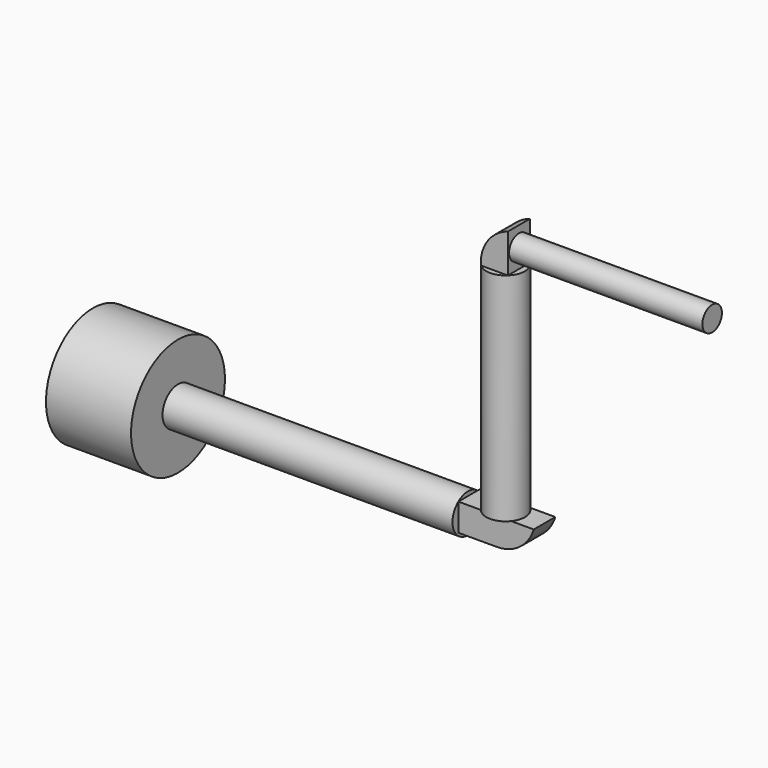
from build123d import *

# Parameters (mm, degrees)
F0_R         = 2.54
F1_DEPTH     = 38.1
F2_W         = 3.5423064731
F2_H         = 3.6002054004
F3_DEPTH     = 9.906
F4_T1_DEPTH  = 27.8407673004
F5_R         = 2.54
F6_DEPTH     = 28.448
F0_R_2       = 7.7136033571
F7_DEPTH     = 11.176
F9_DEPTH     = 5.08
F10_T1_DEPTH = 27.8075265616
F11_R        = 1.605342172
F12_DEPTH    = 25.4


# Not quite as in the source:
# - a fillet or chamfer that OpenCascade refuses, or shapes differently, is made with other operations: its cross-section is extruded or revolved along the edge and cut away or added


with BuildPart() as f1:
    # F0 (on Right) → F1 (new body)
    with BuildSketch(Plane.YZ):
        with Locations((-112.0406836271, 54.1470609605)):
            Circle(F0_R)
    extrude(amount=F1_DEPTH)

    # F2 (on face) → F3 (join)
    with BuildSketch(Plane.YZ.offset(38.1)):
        with Locations((-111.8464542239, 54.3381667436)):
            Rectangle(F2_W, F2_H)
    extrude(amount=F3_DEPTH)

    # F4: fillet of radius 5.08 on 1 edges, made by hand

    # F4_s2 → F4_t1 (cut)
    with BuildSketch(Plane.XZ.offset(97.9260705737)):
        with BuildLine():
            ThreePointArc((43.1463078345, 52.5380640434), (46.1702988592, 53.5361676357), (48.006, 56.1382694438))
            Line((48.006, 56.1382694438), (48.006, 52.5380640434))
            Line((48.006, 52.5380640434), (43.1463078345, 52.5380640434))
        make_face()
    extrude(amount=F4_T1_DEPTH, mode=Mode.SUBTRACT)

    # F5 (on face) → F6 (join)
    with BuildSketch(Plane.XY.offset(56.1382694438)):
        with Locations((43.053, -112.0406836271)):
            Circle(F5_R)
    extrude(amount=F6_DEPTH)

    # F8 (on face) → F9 (join)
    with BuildSketch(Plane.XY.offset(84.5862694438)):
        with BuildLine():
            Line((44.8093679455, -110.2645377603), (41.2372616213, -110.2645377603))
            Line((41.2372616213, -110.2645377603), (41.2372616213, -113.8168294939))
            ThreePointArc((41.2372616213, -113.8168294939), (41.2667054502, -113.8464388103), (41.2966320545, -113.8755600916))
            Line((41.2966320545, -113.8755600916), (44.8093679455, -113.8755600916))
            Line((44.8093679455, -113.8755600916), (44.8093679455, -110.2645377603))
        make_face()
    extrude(amount=F9_DEPTH)

    # F10: fillet of radius 5.08 on 1 edges, made by hand

    # F10_s2 → F10_t1 (cut)
    with BuildSketch(Plane.XZ.offset(98.1369203463)):
        with BuildLine():
            ThreePointArc((41.2372616213, 84.8152224782), (42.2266320932, 87.8273894828), (44.8093679455, 89.6662694438))
            Line((44.8093679455, 89.6662694438), (41.2372616213, 89.6662694438))
            Line((41.2372616213, 89.6662694438), (41.2372616213, 84.8152224782))
        make_face()
    extrude(amount=F10_T1_DEPTH, mode=Mode.SUBTRACT)

    # F11 (on face) → F12 (join)
    with BuildSketch(Plane.YZ.offset(44.8093679455)):
        with Locations((-112.070048926, 87.1262694438)):
            Circle(F11_R)
    extrude(amount=F12_DEPTH)


with BuildPart() as f7:
    # F0 (on Right) → F7 (new body)
    with BuildSketch(Plane.YZ):
        with Locations((-112.0406836271, 54.1470609605)):
            Circle(F0_R_2)
        with Locations((-112.0406836271, 54.1470609605)):
            Circle(F0_R, mode=Mode.SUBTRACT)
    extrude(amount=-F7_DEPTH)


solid = Compound([f1.part, f7.part])
